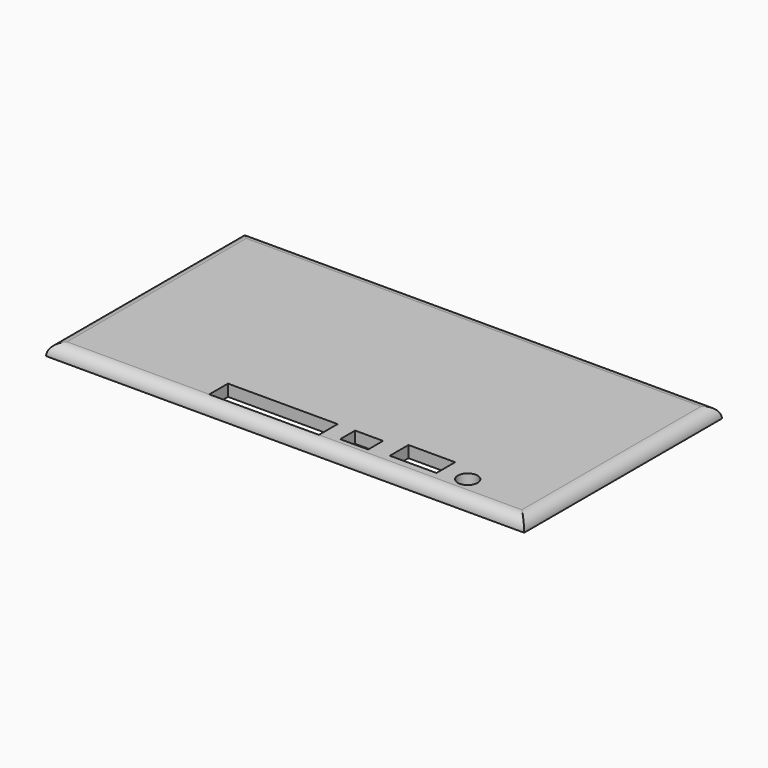
from build123d import *

# Parameters (mm, degrees)
F0_W      = 205
F0_H      = 106
F1_DEPTH  = 5
F2_R      = 4.25
F3_DEPTH  = 500
F4_W      = 20
F4_H      = 10
F5_DEPTH  = 500
F6_W      = 12
F6_H      = 8
F7_DEPTH  = 500
F8_R      = 4.99999
F9_W      = 47
F9_H      = 10
F10_DEPTH = 500


# Not quite as in the source:
# - a fillet or chamfer is up to 0.001 mm smaller than in the source, because OpenCascade refuses the exact size


with BuildPart() as f1:
    # F0 (on Top) → F1 (new body)
    with BuildSketch(Plane.XY):
        with Locations((-719.1119938903, -475.8524597138)):
            Rectangle(F0_W, F0_H)
    extrude(amount=F1_DEPTH)

    # F2 (on face) → F3 (cut)
    with BuildSketch(Plane.XY.offset(5)):
        with Locations((-649.6119938903, -517.8524597138)):
            Circle(F2_R)
    extrude(amount=-F3_DEPTH, mode=Mode.SUBTRACT)

    # F4 (on face) → F5 (cut)
    with BuildSketch(Plane.XY.offset(5)):
        with Locations((-670.6119938903, -515.8524597138)):
            Rectangle(F4_W, F4_H)
    extrude(amount=-F5_DEPTH, mode=Mode.SUBTRACT)

    # F6 (on face) → F7 (cut)
    with BuildSketch(Plane.XY.offset(5)):
        with Locations((-695.1119938903, -517.8524597138)):
            Rectangle(F6_W, F6_H)
    extrude(amount=-F7_DEPTH, mode=Mode.SUBTRACT)

    # F8 (radius 5 in the source; OpenCascade refuses exactly that, so slightly less here)
    f8_edges = [f1.edges().sort_by_distance(p)[0] for p in [
        (-821.611994, -475.85246, 5),
        (-719.111994, -528.85246, 5),
        (-616.611994, -475.85246, 5),
        (-719.111994, -422.85246, 5),
    ]]
    fillet(f8_edges, radius=F8_R)

    # F9 (on face) → F10 (cut)
    with BuildSketch(Plane.XY.offset(5)):
        with Locations((-732.1119938903, -518.8524597138)):
            Rectangle(F9_W, F9_H)
    extrude(amount=-F10_DEPTH, mode=Mode.SUBTRACT)


solid = f1.part
